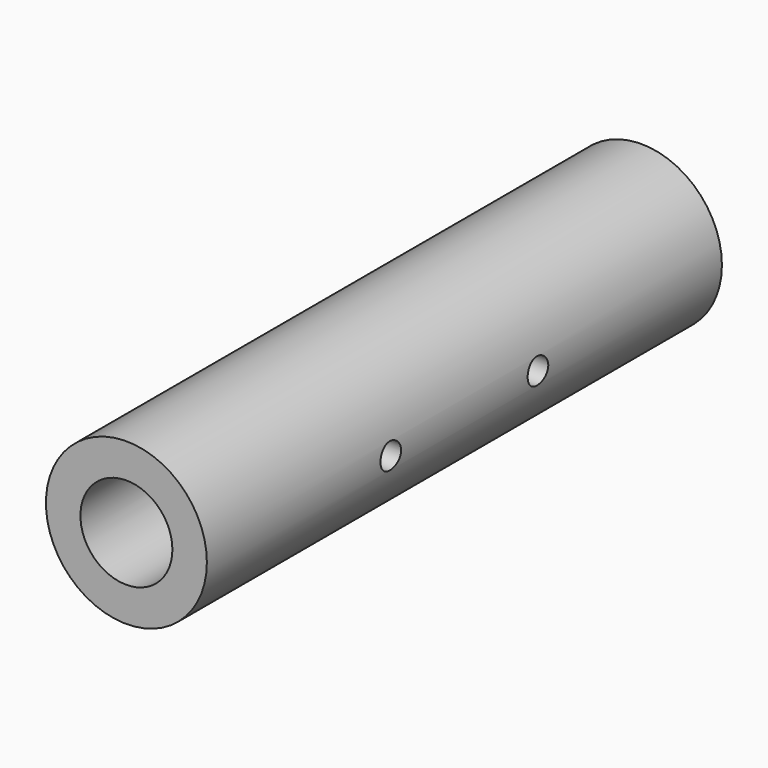
from build123d import *

# Parameters (mm, degrees)
F0_R     = 11.1125
F0_R_2   = 6.35
F1_DEPTH = 44.45
F3_R     = 1.778
F4_DEPTH = 22.226


# Not quite as in the source:
# - a length typed as a fraction of an inch, garbled in the dataset ("3 / 203.2 mm" for 3/8 in), is restored


with BuildPart() as f1:
    # F0 (on Front) → F1 (new body, symmetric)
    with BuildSketch(Plane.XZ):
        Circle(F0_R)
        Circle(F0_R_2, mode=Mode.SUBTRACT)
    extrude(amount=F1_DEPTH, both=True)

    # F3 (on offset) → F4 (cut, through all)
    with BuildSketch(Plane.YZ.offset(11.1125)):
        with Locations((-12.7, 0)):
            Circle(F3_R)
        with Locations((12.7, 0)):
            Circle(F3_R)
    extrude(amount=-F4_DEPTH, mode=Mode.SUBTRACT)


solid = f1.part
